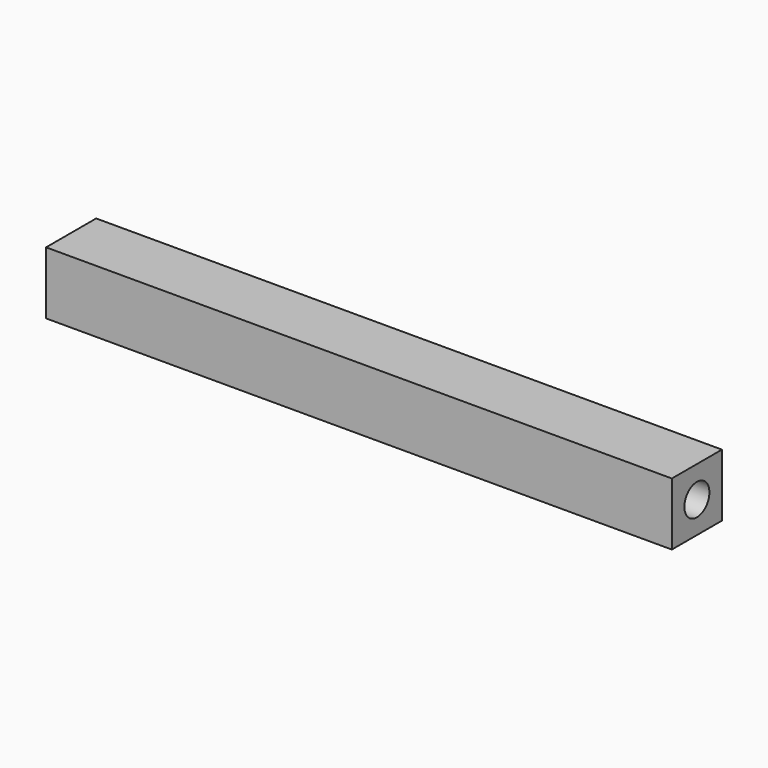
from build123d import *

# Parameters (mm, degrees)
F0_W     = 76.2
F0_H     = 12.7
F1_DEPTH = 12.7
F2_R     = 3.175
F3_DEPTH = 85.27917
F4_DEPTH = 25.4
F5_DEPTH = 25.4


with BuildPart() as f1:
    # F0 (on Top) → F1 (new body)
    with BuildSketch(Plane.XY):
        with Locations((-38.1, -6.35)):
            Rectangle(F0_W, F0_H)
    extrude(amount=-F1_DEPTH)

    # F2 (on face) → F3 (cut)
    with BuildSketch(Plane.YZ):
        with Locations((-6.35, -6.35)):
            Circle(F2_R)
    extrude(amount=-F3_DEPTH, mode=Mode.SUBTRACT)

    # F4 (add): a face of the model
    f4_faces = [f1.faces().sort_by_distance(p)[0] for p in [
        (0, -12.5203948776, -6.35),
    ]]
    extrude(f4_faces, amount=F4_DEPTH)

    # F5 (add): a face of the model
    f5_faces = [f1.faces().sort_by_distance(p)[0] for p in [
        (-76.2, -0.1796051224, -6.35),
    ]]
    extrude(f5_faces, amount=F5_DEPTH)


solid = f1.part
